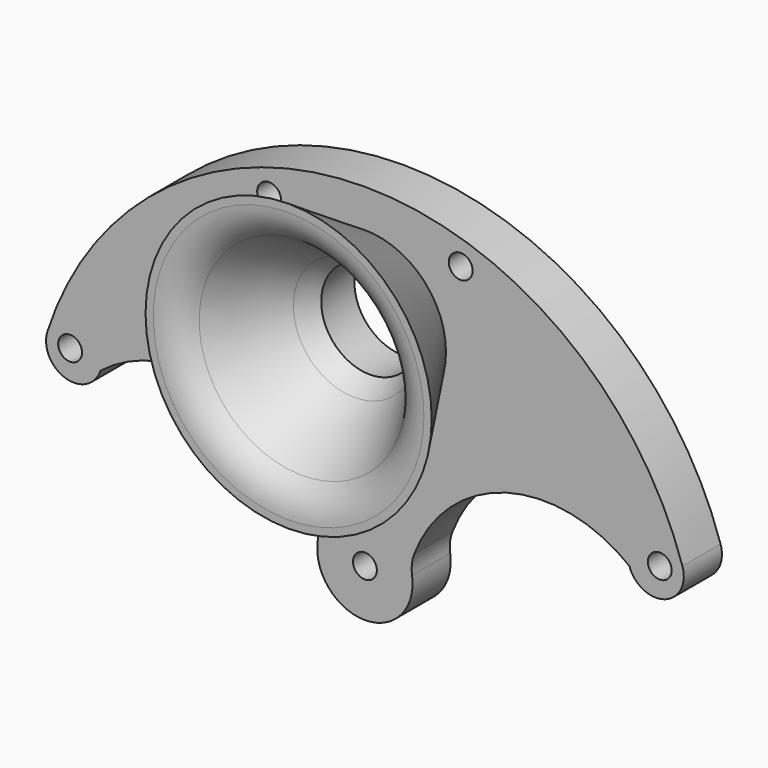
from build123d import *

# Parameters (mm, degrees)
F0_R        = 1.5875
F1_DEPTH    = 6.35
F2_R        = 10.795
F4_R        = 19.05
F6_T        = 3.175
F6_T3_DEPTH = 12.7
F7_R        = 6.477
F8_DEPTH    = 19.051
F9_R        = 5.08


# Not quite as in the source:
# - two fillets or chamfers of one size are made in one step
# - a shell that OpenCascade refuses in one call is made with other operations: the cavity is built on its own and cut out


with BuildPart() as f1:
    # F0 (on Front) → F1 (new body)
    with BuildSketch(Plane.XZ):
        with BuildLine():
            ThreePointArc((35.2153805779, 11.4421707601), (39.8917386836, 9.0594472943), (42.2744621493, 13.7358054))
            ThreePointArc((42.2744621493, 13.7358054), (0, 44.45), (-42.2744621493, 13.7358054))
            ThreePointArc((-42.2744621493, 13.7358054), (-39.8917386836, 9.0594472943), (-35.2153805779, 11.4421707601))
            ThreePointArc((-35.2153805779, 11.4421707601), (-18.0952762982, 14.4949657749), (-6.0392088785, 1.9622579143))
            ThreePointArc((-6.0392088785, 1.9622579143), (0, -6.35), (6.0392088785, 1.9622579143))
            ThreePointArc((6.0392088785, 1.9622579143), (18.0952762982, 14.4949657749), (35.2153805779, 11.4421707601))
        make_face()
        Circle(F0_R, mode=Mode.SUBTRACT)
        with Locations((-39.2548577101, 12.7546764428)):
            Circle(F0_R, mode=Mode.SUBTRACT)
        with Locations((39.2548577101, 12.7546764428)):
            Circle(F0_R, mode=Mode.SUBTRACT)
        with Locations((-12.7546764428, 39.2548577101)):
            Circle(F0_R, mode=Mode.SUBTRACT)
        with Locations((12.7546764428, 39.2548577101)):
            Circle(F0_R, mode=Mode.SUBTRACT)
    extrude(amount=F1_DEPTH)

    # F2 (on face) → F5 section 0
    with BuildSketch(Plane.XZ.offset(6.35)):
        with Locations((0, 28.575)):
            Circle(F2_R)
    # F4 (on offset) → F5 section 1
    with BuildSketch(Plane.XZ.offset(19.05)):
        with Locations((0, 28.575)):
            Circle(F4_R)
    loft()

    # F6: shell of thickness 3.175, made by hand


with BuildPart() as f6_core1:
    # F6_t2: copy of F1
    add(f1.part)

    # the walls: a layer under each face that stays
    f6_faces = [f6_core1.faces().sort_by_distance(p)[0] for p in [
        (18.0952762982, -3.175, 14.4949657749),
        (0, -3.175, -6.35),
        (39.8917386836, -3.175, 9.0594472943),
        (0, 0, 19.05),
        (-28.3040667791, -6.35, 19.05),
        (-18.0952762982, -3.175, 14.4949657749),
        (0, -3.175, 44.45),
        (-39.8917386836, -3.175, 9.0594472943),
        (-1.5875, -3.175, 0),
        (-40.8423577101, -3.175, 12.7546764428),
        (37.6673577101, -3.175, 12.7546764428),
        (-14.3421764428, -3.175, 39.2548577101),
        (11.1671764428, -3.175, 39.2548577101),
        (-14.9225, -12.7, 28.575),
    ]]
    thicken(f6_faces, amount=-F6_T, mode=Mode.SUBTRACT)

    # F6_s4 → F6_t3 (cut)
    with BuildSketch(Plane.XZ.offset(-3.175)):
        Polygon((6.0999585135, 1.9634355139), (2.9838498192, 2.8256269079), (2.7217112336, 1.8979499721), (3.0196044392, 0.9811289571), align=None)
        Polygon((35.1655409151, 11.4074157187), (37.179742419, 13.9365459438), (37.9370918115, 13.3401207322), (38.2349850172, 12.4232997172), align=None)
        Polygon((-6.0999585135, 1.9634355139), (-3.0196044392, 0.9811289571), (-2.7217112336, 1.8979499721), (-2.9838498192, 2.8256269079), align=None)
        Polygon((-35.1655409151, 11.4074157187), (-37.179742419, 13.9365459438), (-37.9370918115, 13.3401207322), (-38.2349850172, 12.4232997172), align=None)
    extrude(amount=F6_T3_DEPTH, mode=Mode.SUBTRACT)

    # F6_s5 → F6_t6 (revolve, cut)
    with BuildSketch(Plane.XY.offset(28.575)):
        Polygon((10.8216205848, -6.3644466199), (10.795, -3.175), (4.9444718097, -3.175), (8.1329415182, -8.0803380131), align=None)
    revolve(axis=Axis((0, -6.35, 28.575), (0, -1, 0)), mode=Mode.SUBTRACT)


with BuildPart() as f1_1:
    add(f1.part)

    # what is left inside the walls is the cavity
    f6_cavity = [f6_core1.part.solids().sort_by_distance(p)[0] for p in [
        (-10.483081, -11.754195, 28.575),
    ]]
    add(f6_cavity, mode=Mode.SUBTRACT)

    # F7 (on face) → F8 (cut, through all)
    with BuildSketch(Plane.XZ.offset(19.05)):
        with Locations((0, 28.575)):
            Circle(F7_R)
    extrude(amount=-F8_DEPTH, mode=Mode.SUBTRACT)

    # F9
    f9_edges = [f1_1.edges().sort_by_distance(p)[0] for p in [
        (6.039209, -3.175, 1.962258),
        (-6.039209, -3.175, 1.962258),
        (-15.263222, -19.05, 28.575),
    ]]
    fillet(f9_edges, radius=F9_R)


solid = f1_1.part
